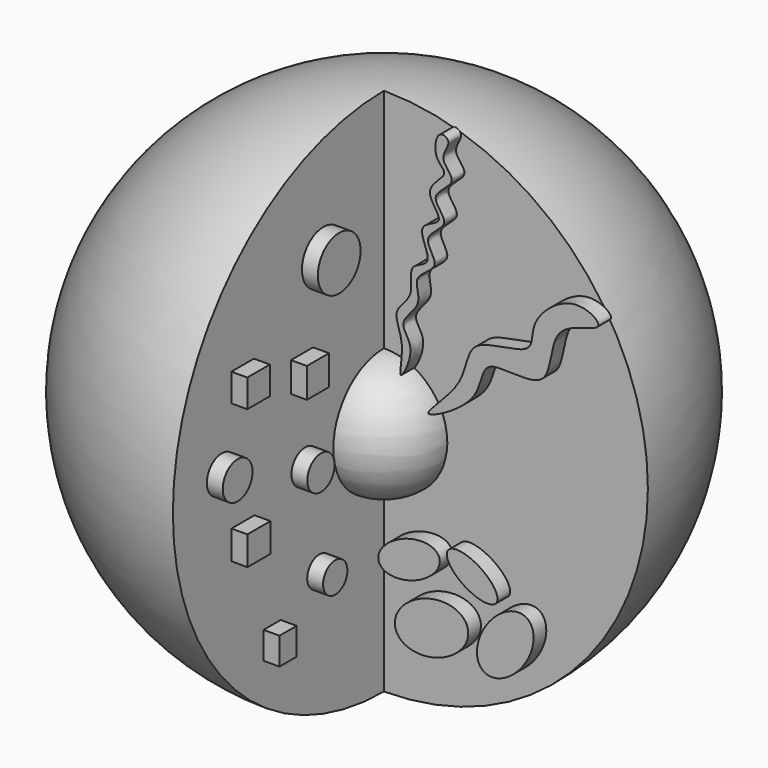
from build123d import *

# Parameters (mm, degrees)
F1_ANGLE  = 270
F5_DEPTH  = 1.5
F7_DEPTH  = 1.5
F9_DEPTH  = 1.5
F11_DEPTH = 1.5
F13_DEPTH = 1.5
F15_DEPTH = 1.5
F16_W     = 2.0231939852
F16_H     = 2.5716638193
F17_DEPTH = 1.5
F18_W     = 2.7137994766
F18_H     = 2.726720646
F19_DEPTH = 1.5
F20_W     = 2.6141293347
F20_H     = 2.8187632561
F21_DEPTH = 1.5
F22_W     = 2.6620849967
F22_H     = 2.6391372085
F23_DEPTH = 1.5
F24_R     = 1.4370007645
F25_DEPTH = 1.5
F26_R     = 1.6153418838
F27_DEPTH = 1.5
F28_R     = 2.5244050993
F29_DEPTH = 1.5
F30_R     = 1.7591343941
F31_DEPTH = 1.5


with BuildPart() as f1:
    # F0 (on Front) → F1 (revolve)
    with BuildSketch(Plane.XZ):
        with BuildLine():
            Line((0, 50), (0, 0))
            ThreePointArc((0, 0), (24.941704642, 25), (0, 50))
        make_face()
    revolve(axis=Axis((0, 0, 25), (0, 0, 1)), revolution_arc=F1_ANGLE)


with BuildPart() as f3:
    # F2 (on Right) → F3 (revolve)
    with BuildSketch(Plane.YZ):
        with BuildLine():
            Line((0, 28.5625886172), (0, 16.7574677616))
            ThreePointArc((0, 16.7574677616), (5.9820465661, 22.6600281894), (0, 28.5625886172))
        make_face()
    revolve(axis=Axis((0, 0, 25), (0, 0, 1)))


with BuildPart() as f5:
    # F4 (on face) → F5 (new body)
    with BuildSketch(Plane.XZ):
        with BuildLine():
            add(Edge.make_bspline(
                [(2.7956720442, 27.8470981866), (2.9904627952, 27.8448492764), (4.4394987788, 30.6193332149), (2.1596972389, 32.2268383068), (5.1422043681, 34.264529425), (3.5867407266, 36.6397632213), (6.9634816182, 37.8791494485), (4.3398564506, 40.2065305241), (7.9720860251, 41.7472661522), (4.9878929449, 43.818820989), (8.614943398, 45.4801712033), (6.1152501035, 47.0790492461), (7.7862925241, 48.7292660883), (6.1857063252, 49.5894589331), (5.7669194082, 46.8347071409), (7.6742571502, 45.9692564425), (4.4346146602, 44.1174115987), (7.4731429266, 41.6173241233), (3.7706683482, 41.1665389827), (6.2522912482, 37.7862702109), (3.2448278517, 37.539179235), (4.2949109783, 34.6882676012), (1.7028003495, 33.0674446361), (3.3457190168, 30.7592846364), (2.6029034227, 27.8493237509), (2.7956720442, 27.8470981866)],
                knots=[0, 0, 0, 0, 0.0487164199, 0.0918818852, 0.1400450271, 0.1829024321, 0.2285271846, 0.2714480804, 0.3179415848, 0.360395211, 0.4068888, 0.447026121, 0.4855744397, 0.5130928087, 0.5562777323, 0.5910238539, 0.6371760903, 0.6823644721, 0.7240283638, 0.7725467188, 0.8118178904, 0.8572034241, 0.9029190479, 0.951789307, 1, 1, 1, 1], degree=3))
        make_face()
    extrude(amount=F5_DEPTH)


with BuildPart() as f7:
    # F6 (on face) → F7 (new body)
    with BuildSketch(Plane.XZ):
        with BuildLine():
            add(Edge.make_bspline(
                [(5.397609435, 25.5058333278), (5.6220965883, 25.2766681782), (10.7839998717, 27.8247844169), (10.0424494126, 32.478465447), (17.6037468849, 30.1908646739), (16.3745709476, 37.3427854343), (22.9607435954, 37.5133872437), (19.0554981673, 40.1080300578), (14.7235807428, 36.5026213563), (15.7267199542, 33.2338279485), (8.7376836433, 33.4876088459), (9.335550697, 29.0083497706), (5.1831310874, 25.7247811022), (5.397609435, 25.5058333278)],
                knots=[0, 0, 0, 0, 0.1007013141, 0.1855574915, 0.2855290562, 0.3853154809, 0.4748692985, 0.542805581, 0.6433085131, 0.7125446398, 0.8131138445, 0.9037884746, 1, 1, 1, 1], degree=3))
        make_face()
    extrude(amount=F7_DEPTH)


with BuildPart() as f9:
    # F8 (on face) → F9 (new body)
    with BuildSketch(Plane.XZ):
        with BuildLine():
            add(Edge.make_bspline(
                [(9.065805003, 9.0021379292), (7.6473033774, 12.8049250519), (3.2987350026, 9.0168824333), (-1.0498333722, 5.2288398147), (4.7172366282, 5.2140953106), (10.4843066287, 5.1993508065), (9.065805003, 9.0021379292)],
                knots=[0, 0, 0, 2.0943951024, 2.0943951024, 4.1887902048, 4.1887902048, 6.2831853072, 6.2831853072, 6.2831853072], degree=2, weights=[1, 0.5, 1, 0.5, 1, 0.5, 1]))
        make_face()
    extrude(amount=F9_DEPTH)


with BuildPart() as f11:
    # F10 (on face) → F11 (new body)
    with BuildSketch(Plane.XZ):
        with BuildLine():
            add(Edge.make_bspline(
                [(14.75676056, 11.4624239504), (11.865391693, 13.5915475804), (10.1695639635, 8.260784247), (8.473736234, 2.9300209135), (13.0609328305, 6.131660617), (17.648129427, 9.3333003204), (14.75676056, 11.4624239504)],
                knots=[0, 0, 0, 2.0943951024, 2.0943951024, 4.1887902048, 4.1887902048, 6.2831853072, 6.2831853072, 6.2831853072], degree=2, weights=[1, 0.5, 1, 0.5, 1, 0.5, 1]))
        make_face()
    extrude(amount=F11_DEPTH)


with BuildPart() as f13:
    # F12 (on face) → F13 (new body)
    with BuildSketch(Plane.XZ):
        with BuildLine():
            add(Edge.make_bspline(
                [(6.406606175, 13.8894356787), (5.3475402918, 16.5385683784), (1.6153357768, 13.5102516865), (-2.1168687381, 10.4819349945), (2.6744016601, 10.8611189867), (7.4656720582, 11.240302979), (6.406606175, 13.8894356787)],
                knots=[0, 0, 0, 2.0943951024, 2.0943951024, 4.1887902048, 4.1887902048, 6.2831853072, 6.2831853072, 6.2831853072], degree=2, weights=[1, 0.5, 1, 0.5, 1, 0.5, 1]))
        make_face()
    extrude(amount=F13_DEPTH)


with BuildPart() as f15:
    # F14 (on face) → F15 (new body)
    with BuildSketch(Plane.XZ):
        with BuildLine():
            add(Edge.make_bspline(
                [(11.8345357478, 11.8562486023), (12.9630766276, 13.6919215926), (8.9418355109, 14.8993725259), (4.9205943942, 16.1068234593), (7.8132946311, 13.0636995356), (10.7059948679, 10.0205756119), (11.8345357478, 11.8562486023)],
                knots=[0, 0, 0, 2.0943951024, 2.0943951024, 4.1887902048, 4.1887902048, 6.2831853072, 6.2831853072, 6.2831853072], degree=2, weights=[1, 0.5, 1, 0.5, 1, 0.5, 1]))
        make_face()
    extrude(amount=F15_DEPTH)


with BuildPart() as f17:
    # F16 (on face) → F17 (new body)
    with BuildSketch(Plane.YZ):
        with Locations((-13.2142771035, 9.6330610104)):
            Rectangle(F16_W, F16_H)
    extrude(amount=F17_DEPTH)


with BuildPart() as f19:
    # F18 (on face) → F19 (new body)
    with BuildSketch(Plane.YZ):
        with Locations((-16.6557505727, 19.5278087631)):
            Rectangle(F18_W, F18_H)
    extrude(amount=F19_DEPTH)


with BuildPart() as f21:
    # F20 (on face) → F21 (new body)
    with BuildSketch(Plane.YZ):
        with Locations((-9.6845645458, 30.6384302676)):
            Rectangle(F20_W, F20_H)
    extrude(amount=F21_DEPTH)


with BuildPart() as f23:
    # F22 (on face) → F23 (new body)
    with BuildSketch(Plane.YZ):
        with Locations((-16.6983343661, 32.6275713742)):
            Rectangle(F22_W, F22_H)
    extrude(amount=F23_DEPTH)


with BuildPart() as f25:
    # F24 (on face) → F25 (new body)
    with BuildSketch(Plane.YZ):
        with Locations((-7.6350085437, 13.0909802392)):
            Circle(F24_R)
    extrude(amount=F25_DEPTH)


with BuildPart() as f27:
    # F26 (on face) → F27 (new body)
    with BuildSketch(Plane.YZ):
        with Locations((-9.3197263777, 22.4967859685)):
            Circle(F26_R)
    extrude(amount=F27_DEPTH)


with BuildPart() as f29:
    # F28 (on face) → F29 (new body)
    with BuildSketch(Plane.YZ):
        with Locations((-7.1682855487, 39.051450789)):
            Circle(F28_R)
    extrude(amount=F29_DEPTH)


with BuildPart() as f31:
    # F30 (on face) → F31 (new body)
    with BuildSketch(Plane.YZ):
        with Locations((-19.1661678255, 25.8615706116)):
            Circle(F30_R)
    extrude(amount=F31_DEPTH)


solid = Compound([f1.part, f3.part, f5.part, f7.part, f9.part, f11.part, f13.part, f15.part, f17.part, f19.part, f21.part, f23.part, f25.part, f27.part, f29.part, f31.part])
